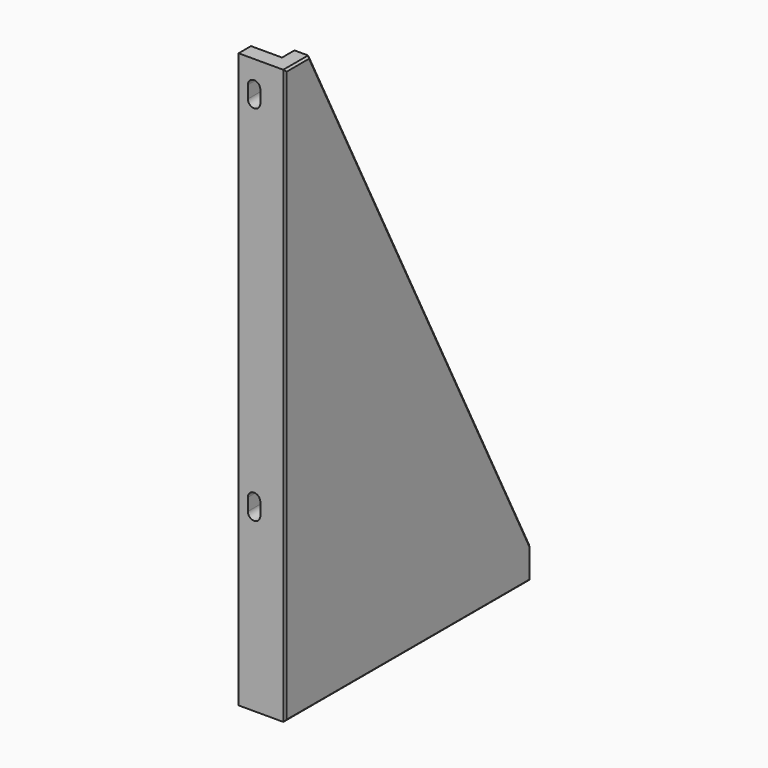
from build123d import *

# Parameters (mm, degrees)
F0_W        = 54
F0_H        = 5
F0_W_2      = 40
F1_DEPTH    = 5
F2_DEPTH    = 10
F3_DEPTH    = 35
F5_DEPTH    = 5.001
F7_DEPTH    = 5.001
F4_W        = 35
F4_H        = 4
F8_DEPTH    = 40
F9_T4_DEPTH = 106.8673195186
F10_R       = 2
F11_R       = 10
F12_SIZE    = 0.6


# Not quite as in the source:
# - a fillet or chamfer that OpenCascade refuses, or shapes differently, is made with other operations: its cross-section is extruded or revolved along the edge and cut away or added


with BuildPart() as f1:
    # F0 (on Right) → F1 (new body)
    with BuildSketch(Plane.YZ):
        Polygon((0, 185), (0, 0), (5, 0), (5, 5), (5, 185), align=None)
        with Locations((32, 2.5)):
            Rectangle(F0_W, F0_H)
        Polygon((10, 185), (5, 185), (5, 5), (59, 5), (99, 5), (99, 10), align=None)
        with Locations((79, 2.5)):
            Rectangle(F0_W_2, F0_H)
    extrude(amount=F1_DEPTH)

    # F0 (on Right) → F2 (join)
    with BuildSketch(Plane.YZ):
        Polygon((0, 185), (0, 0), (5, 0), (5, 5), (5, 185), align=None)
    extrude(amount=-F2_DEPTH)

    # F0 (on Right) → F3 (join)
    with BuildSketch(Plane.YZ):
        with Locations((79, 2.5)):
            Rectangle(F0_W_2, F0_H)
    extrude(amount=-F3_DEPTH)

    # F4 (on face) → F5 (cut, through all)
    with BuildSketch(Plane.XY.offset(5)):
        with BuildLine():
            Line((-26.05, 69), (-26.05, 71))
            ThreePointArc((-26.05, 71), (-27.8, 72.75), (-29.55, 71))
            Line((-29.55, 71), (-29.55, 69))
            Line((-29.55, 69), (-29.55, 67))
            ThreePointArc((-29.55, 67), (-27.8, 65.25), (-26.05, 67))
            Line((-26.05, 67), (-26.05, 69))
        make_face()
        with BuildLine():
            Line((-26.05, 89), (-26.05, 91))
            ThreePointArc((-26.05, 91), (-27.8, 92.75), (-29.55, 91))
            Line((-29.55, 91), (-29.55, 89))
            Line((-29.55, 89), (-29.55, 87))
            ThreePointArc((-29.55, 87), (-27.8, 85.25), (-26.05, 87))
            Line((-26.05, 87), (-26.05, 89))
        make_face()
    extrude(amount=-F5_DEPTH, mode=Mode.SUBTRACT)

    # F6 (on face) → F7 (cut, through all)
    with BuildSketch(Plane(origin=(0, 5, 0), x_dir=(-1, 0, 0), z_dir=(0, 1, 0))):
        with BuildLine():
            Line((7, 58), (7, 60))
            ThreePointArc((7, 60), (5, 62), (3, 60))
            Line((3, 60), (3, 58))
            Line((3, 58), (3, 56))
            ThreePointArc((3, 56), (5, 54), (7, 56))
            Line((7, 56), (7, 58))
        make_face()
        with BuildLine():
            Line((7, 175), (7, 177))
            ThreePointArc((7, 177), (5, 179), (3, 177))
            Line((3, 177), (3, 175))
            Line((3, 175), (3, 173))
            ThreePointArc((3, 173), (5, 171), (7, 173))
            Line((7, 173), (7, 175))
        make_face()
    extrude(amount=-F7_DEPTH, mode=Mode.SUBTRACT)

    # F4 (on face) → F8 (join)
    with BuildSketch(Plane.XY.offset(5)):
        with Locations((-17.5, 79)):
            Rectangle(F4_W, F4_H)
    extrude(amount=F8_DEPTH)

    # F9: chamfer of 40 on 1 edges, made by hand


with BuildPart() as f9_tool2:
    # F9_s3 → F9_t4 (new body)
    with BuildSketch(Plane.XZ.offset(-183.8673195186)):
        Polygon((-35, 5), (5, 45), (-35, 45), align=None)
    extrude(amount=F9_T4_DEPTH)

    split(bisect_by=Plane.YZ, keep=Keep.BOTTOM)


with BuildPart() as f1_1:
    add(f1.part)

    # F9_t1: cut F9_tool2
    add(f9_tool2.part, mode=Mode.SUBTRACT)

    # F10
    f10_edges = [f1_1.edges().sort_by_distance(p)[0] for p in [
        (-17.5, 77, 5),
        (0, 77, 22.5),
        (0, 81, 22.5),
        (-17.5, 81, 5),
        (0, 68, 5),
        (0, 90, 5),
    ]]
    fillet(f10_edges, radius=F10_R)

    # F11
    f11_edges = [f1_1.edges().sort_by_distance(p)[0] for p in [
        (-35, 59, 2.5),
        (-35, 99, 2.5),
    ]]
    fillet(f11_edges, radius=F11_R)

    # F12
    f12_edges = [f1_1.edges().sort_by_distance(p)[0] for p in [
        (5, 0, 92.5),
        (5, 49.5, 0),
        (5, 99, 5),
        (5, 54.5, 97.5),
        (5, 5, 185),
    ]]
    chamfer(f12_edges, length=F12_SIZE)


solid = f1_1.part
